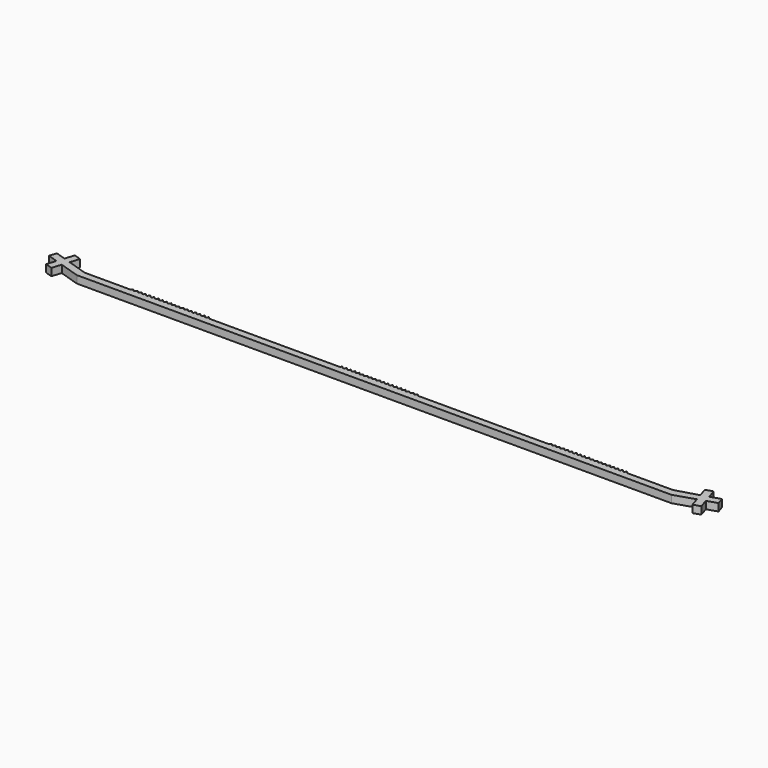
from build123d import *

# Parameters (mm, degrees)
F1_DEPTH = 4.45


# Not quite as in the source:
# - ends of sketch curves that miss each other by under 0.0002 mm in the source are joined


with BuildPart() as f1:
    # F0 (on Top) → F1 (new body)
    with BuildSketch(Plane.XY):
        Polygon((-331.4450657695, 32.3000406861), (-319.3518902557, 28.4212385525), (36.2481097443, 28.4212385525), (48.3412852582, 32.3000401984), (50.1221609735, 26.7476964974), (54.3595334961, 28.1068043316), (52.5786563237, 33.6591525753), (58.6252440806, 35.5985536421), (57.2661362464, 39.8359261646), (51.2195484895, 37.8965250978), (49.4386591004, 43.4489114302), (45.2012865779, 42.089803596), (46.9821759669, 36.5374172636), (33.7284139879, 32.6586156178), (6.2338030338, 32.6586156178), (5.3678165293, 33.8001064959), (4.5018300192, 32.6586156178), (3.7338030338, 32.6586156178), (2.8678165293, 33.8001064959), (2.0018300192, 32.6586156178), (1.2338030338, 32.6586156178), (0.3678165293, 33.8001064959), (-0.4981699808, 32.6586156178), (-1.2661969662, 32.6586156178), (-2.1321834707, 33.8001064959), (-2.9981699808, 32.6586156178), (-3.7661969662, 32.6586156178), (-4.6321834707, 33.8001064959), (-5.4981699808, 32.6586156178), (-6.2661969662, 32.6586156178), (-7.1321834707, 33.8001064959), (-7.9981699808, 32.6586156178), (-8.7661969662, 32.6586156178), (-9.6321834707, 33.8001064959), (-10.4981699808, 32.6586156178), (-11.2661969662, 32.6586156178), (-12.1321834707, 33.8001064959), (-12.9981699808, 32.6586156178), (-13.7661969662, 32.6586156178), (-14.6321834707, 33.8001064959), (-15.4981699808, 32.6586156178), (-16.2661969662, 32.6586156178), (-17.1321834707, 33.8001064959), (-17.9981699808, 32.6586156178), (-18.7661969662, 32.6586156178), (-19.6321834707, 33.8001064959), (-20.4981699808, 32.6586156178), (-21.2661969662, 32.6586156178), (-22.1321834707, 33.8001064959), (-22.9981699808, 32.6586156178), (-23.7661969662, 32.6586156178), (-24.6321834707, 33.8001064959), (-25.4981699808, 32.6586156178), (-26.2661969662, 32.6586156178), (-27.1321834707, 33.8001064959), (-27.9981699808, 32.6586156178), (-28.7661969662, 32.6586156178), (-29.6321834707, 33.8001064959), (-30.4981699808, 32.6586156178), (-31.2661969662, 32.6586156178), (-32.1321834707, 33.8001064959), (-32.9981699808, 32.6586156178), (-33.7661969662, 32.6586156178), (-34.6321834707, 33.8001064959), (-35.4981699808, 32.6586156178), (-36.2661969662, 32.6586156178), (-37.1321834707, 33.8001064959), (-37.9981699808, 32.6586156178), (-38.7661969662, 32.6586156178), (-39.6321834707, 33.8001064959), (-40.4981699808, 32.6586156178), (-118.7661969662, 32.6586156178), (-119.6321834707, 33.8001064959), (-120.4981699808, 32.6586156178), (-121.2661969662, 32.6586156178), (-122.1321834707, 33.8001064959), (-122.9981699808, 32.6586156178), (-123.7661969662, 32.6586156178), (-124.6321834707, 33.8001064959), (-125.4981699808, 32.6586156178), (-126.2661969662, 32.6586156178), (-127.1321834707, 33.8001064959), (-127.9981699808, 32.6586156178), (-128.7661969662, 32.6586156178), (-129.6321834707, 33.8001064959), (-130.4981699808, 32.6586156178), (-131.2661969662, 32.6586156178), (-132.1321834707, 33.8001064959), (-132.9981699808, 32.6586156178), (-133.7661969662, 32.6586156178), (-134.6321834707, 33.8001064959), (-135.4981699808, 32.6586156178), (-136.2661969662, 32.6586156178), (-137.1321834707, 33.8001064959), (-137.9981699808, 32.6586156178), (-138.7661969662, 32.6586156178), (-139.6321834707, 33.8001064959), (-140.4981699808, 32.6586156178), (-141.2661969662, 32.6586156178), (-142.1321834707, 33.8001064959), (-142.9981699808, 32.6586156178), (-143.7661969662, 32.6586156178), (-144.6321834707, 33.8001064959), (-145.4981699808, 32.6586156178), (-146.2661969662, 32.6586156178), (-147.1321834707, 33.8001064959), (-147.9981699808, 32.6586156178), (-148.7661969662, 32.6586156178), (-149.6321834707, 33.8001064959), (-150.4981699808, 32.6586156178), (-151.2661969662, 32.6586156178), (-152.1321834707, 33.8001064959), (-152.9981699808, 32.6586156178), (-153.7661969662, 32.6586156178), (-154.6321834707, 33.8001064959), (-155.4981699808, 32.6586156178), (-156.2661969662, 32.6586156178), (-157.1321834707, 33.8001064959), (-157.9981699808, 32.6586156178), (-158.7661969662, 32.6586156178), (-159.6321834707, 33.8001064959), (-160.4981699808, 32.6586156178), (-161.2661969662, 32.6586156178), (-162.1321834707, 33.8001064959), (-162.9981699808, 32.6586156178), (-163.7661969662, 32.6586156178), (-164.6321834707, 33.8001064959), (-165.4981699808, 32.6586156178), (-243.7661969662, 32.6586156178), (-244.6321834707, 33.8001064959), (-245.4981699808, 32.6586156178), (-246.2661969662, 32.6586156178), (-247.1321834707, 33.8001064959), (-247.9981699808, 32.6586156178), (-248.7661969662, 32.6586156178), (-249.6321834707, 33.8001064959), (-250.4981699808, 32.6586156178), (-251.2661969662, 32.6586156178), (-252.1321834707, 33.8001064959), (-252.9981699808, 32.6586156178), (-253.7661969662, 32.6586156178), (-254.6321834707, 33.8001064959), (-255.4981699808, 32.6586156178), (-256.2661969662, 32.6586156178), (-257.1321834707, 33.8001064959), (-257.9981699808, 32.6586156178), (-258.7661969662, 32.6586156178), (-259.6321834707, 33.8001064959), (-260.4981699808, 32.6586156178), (-261.2661969662, 32.6586156178), (-262.1321834707, 33.8001064959), (-262.9981699808, 32.6586156178), (-263.7661969662, 32.6586156178), (-264.6321834707, 33.8001064959), (-265.4981699808, 32.6586156178), (-266.2661969662, 32.6586156178), (-267.1321834707, 33.8001064959), (-267.9981699808, 32.6586156178), (-268.7661969662, 32.6586156178), (-269.6321834707, 33.8001064959), (-270.4981699808, 32.6586156178), (-271.2661969662, 32.6586156178), (-272.1321834707, 33.8001064959), (-272.9981699808, 32.6586156178), (-273.7661969662, 32.6586156178), (-274.6321834707, 33.8001064959), (-275.4981699808, 32.6586156178), (-276.2661969662, 32.6586156178), (-277.1321834707, 33.8001064959), (-277.9981699808, 32.6586156178), (-278.7661969662, 32.6586156178), (-279.6321834707, 33.8001064959), (-280.4981699808, 32.6586156178), (-281.2661969662, 32.6586156178), (-282.1321834707, 33.8001064959), (-282.9981699808, 32.6586156178), (-283.7661969662, 32.6586156178), (-284.6321834707, 33.8001064959), (-285.4981699808, 32.6586156178), (-286.2661969662, 32.6586156178), (-287.1321834707, 33.8001064959), (-287.9981699808, 32.6586156178), (-288.7661969662, 32.6586156178), (-289.6321834707, 33.8001064959), (-290.4981699808, 32.6586156178), (-317.9927809644, 32.6586156178), (-330.0859564782, 36.5374177514), (-328.3050670892, 42.0898040837), (-332.5424396117, 43.448911918), (-334.3233290008, 37.8965255856), (-340.3699167577, 39.8359266524), (-341.7290245919, 35.5985541298), (-335.682436835, 33.659153063), (-337.4633140074, 28.1068048194), (-333.2259414848, 26.7476969852), align=None)
    extrude(amount=F1_DEPTH)


solid = f1.part
